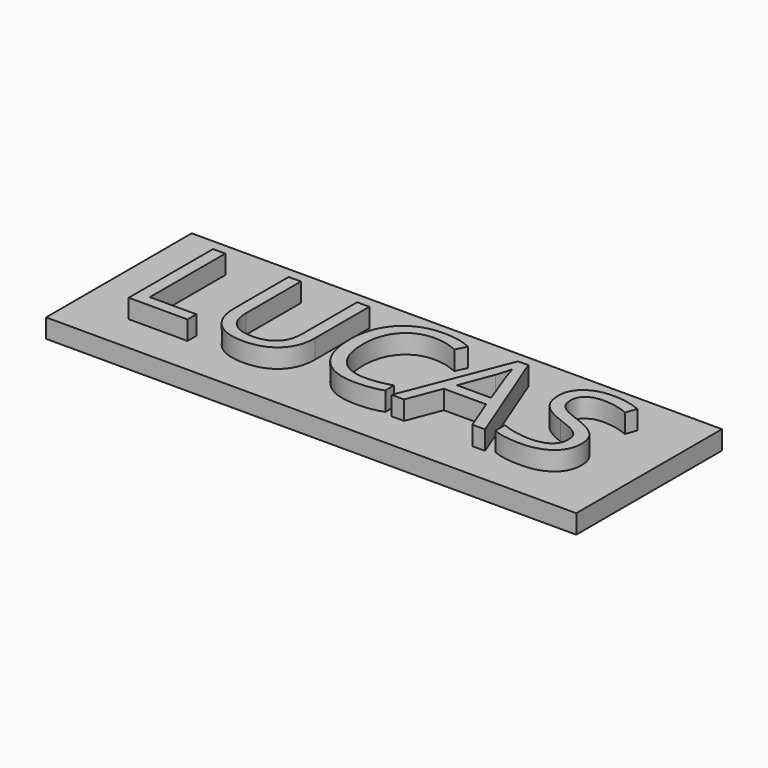
from build123d import *

# Parameters (mm, degrees)
F0_TEXT_SIZE = 24.7679024886
F1_DEPTH     = 6.35
F0_W         = 88.9
F0_H         = 30.5308
F2_DEPTH     = 3.175


# Not quite as in the source:
# - Text() gives the source's letters only with a copy of the font that has no kerning and outlines rounded to 1/6400 em; it was checked with that copy


with BuildPart() as f1:
    # F0 (on Top) → F1 (new body)
    with BuildSketch(Plane.XY):
        with Locations((0, -17.8328897918)):
            Text('LUCAS', F0_TEXT_SIZE, font='Open Sans', text_align=(TextAlign.LEFT, TextAlign.BOTTOM))
    extrude(amount=F1_DEPTH)


with BuildPart() as f2:
    # F0 (on Top) → F2 (new body)
    with BuildSketch(Plane.XY):
        with Locations((38.1, -8.9154)):
            Rectangle(F0_W, F0_H)
        Polygon((12.2872016252, -17.8328897918), (2.4303504317, -17.8328897918), (2.4303504317, -0.1509294058), (4.4853123413, -0.1509294058), (4.4853123413, -15.9714271204), (12.2872016252, -15.9714271204), align=None, mode=Mode.SUBTRACT)
        with BuildLine():
            Line((26.5829253428, -0.1509294058), (28.6378872524, -0.1509294058))
            Line((28.6378872524, -0.1509294058), (28.6378872524, -11.5906043677))
            add(Edge.make_bspline(
                [(28.6378872524, -11.5906043677), (28.6378872524, -14.616932453), (26.8112544439, -16.3468156425)],
                knots=[0, 0, 0, 1, 1, 1], degree=2))
            add(Edge.make_bspline(
                [(26.8112544439, -16.3468156425), (24.9846216353, -18.0766988319), (21.7918842052, -18.0766988319)],
                knots=[0, 0, 0, 1, 1, 1], degree=2))
            add(Edge.make_bspline(
                [(21.7918842052, -18.0766988319), (18.599146775, -18.0766988319), (16.8518486541, -16.3332706958)],
                knots=[0, 0, 0, 1, 1, 1], degree=2))
            add(Edge.make_bspline(
                [(16.8518486541, -16.3332706958), (15.1045505333, -14.5898425597), (15.1045505333, -11.5441645505)],
                knots=[0, 0, 0, 1, 1, 1], degree=2))
            Line((15.1045505333, -11.5441645505), (15.1045505333, -0.1509294058))
            Line((15.1045505333, -0.1509294058), (17.1633824276, -0.1509294058))
            Line((17.1633824276, -0.1509294058), (17.1633824276, -11.6873539868))
            add(Edge.make_bspline(
                [(17.1633824276, -11.6873539868), (17.1633824276, -13.9009852717), (18.3727526663, -15.0871356018)],
                knots=[0, 0, 0, 1, 1, 1], degree=2))
            add(Edge.make_bspline(
                [(18.3727526663, -15.0871356018), (19.582122905, -16.2732859319), (21.9273336719, -16.2732859319)],
                knots=[0, 0, 0, 1, 1, 1], degree=2))
            add(Edge.make_bspline(
                [(21.9273336719, -16.2732859319), (24.1641848654, -16.2732859319), (25.3735551041, -15.0813306247)],
                knots=[0, 0, 0, 1, 1, 1], degree=2))
            add(Edge.make_bspline(
                [(25.3735551041, -15.0813306247), (26.5829253428, -13.8893753174), (26.5829253428, -11.6641340782)],
                knots=[0, 0, 0, 1, 1, 1], degree=2))
            Line((26.5829253428, -11.6641340782), (26.5829253428, -0.1509294058))
        make_face(mode=Mode.SUBTRACT)
        with BuildLine():
            add(Edge.make_bspline(
                [(44.9034332148, -2.6780294566), (42.8949111224, -1.737623159), (40.88638903, -1.737623159)],
                knots=[0, 0, 0, 1, 1, 1], degree=2))
            add(Edge.make_bspline(
                [(40.88638903, -1.737623159), (37.9722905028, -1.737623159), (36.2849771458, -3.678420518)],
                knots=[0, 0, 0, 1, 1, 1], degree=2))
            add(Edge.make_bspline(
                [(36.2849771458, -3.678420518), (34.5976637887, -5.6192178771), (34.5976637887, -8.9938445912)],
                knots=[0, 0, 0, 1, 1, 1], degree=2))
            add(Edge.make_bspline(
                [(34.5976637887, -8.9938445912), (34.5976637887, -12.4613509396), (36.2249923819, -14.3557084815)],
                knots=[0, 0, 0, 1, 1, 1], degree=2))
            add(Edge.make_bspline(
                [(36.2249923819, -14.3557084815), (37.8523209751, -16.2500660234), (40.8631691214, -16.2500660234)],
                knots=[0, 0, 0, 1, 1, 1], degree=2))
            add(Edge.make_bspline(
                [(40.8631691214, -16.2500660234), (42.7130218385, -16.2500660234), (45.0853224987, -15.584428644)],
                knots=[0, 0, 0, 1, 1, 1], degree=2))
            Line((45.0853224987, -15.584428644), (45.0853224987, -17.3839715592))
            add(Edge.make_bspline(
                [(45.0853224987, -17.3839715592), (43.2470797359, -18.0766988319), (40.5497003555, -18.0766988319)],
                knots=[0, 0, 0, 1, 1, 1], degree=2))
            add(Edge.make_bspline(
                [(40.5497003555, -18.0766988319), (36.6448857288, -18.0766988319), (34.5221990858, -15.7043981717)],
                knots=[0, 0, 0, 1, 1, 1], degree=2))
            add(Edge.make_bspline(
                [(34.5221990858, -15.7043981717), (32.3995124429, -13.3320975114), (32.3995124429, -8.9667546978)],
                knots=[0, 0, 0, 1, 1, 1], degree=2))
            add(Edge.make_bspline(
                [(32.3995124429, -8.9667546978), (32.3995124429, -6.2345454545), (33.4211884205, -4.1795835449)],
                knots=[0, 0, 0, 1, 1, 1], degree=2))
            add(Edge.make_bspline(
                [(33.4211884205, -4.1795835449), (34.4428643982, -2.1246216353), (36.3720518029, -1.0120010157)],
                knots=[0, 0, 0, 1, 1, 1], degree=2))
            add(Edge.make_bspline(
                [(36.3720518029, -1.0120010157), (38.3012392077, 0.1006196039), (40.9134789233, 0.1006196039)],
                knots=[0, 0, 0, 1, 1, 1], degree=2))
            add(Edge.make_bspline(
                [(40.9134789233, 0.1006196039), (43.6921279837, 0.1006196039), (45.7741797867, -0.9133164043)],
                knots=[0, 0, 0, 1, 1, 1], degree=2))
            Line((45.7741797867, -0.9133164043), (44.9034332148, -2.6780294566))
        make_face(mode=Mode.SUBTRACT)
        Polygon((62.1867851701, -17.8328897918), (60.05829355, -17.8328897918), (57.8562722194, -12.2098019299), (50.7703301168, -12.2098019299), (48.5953986795, -17.8328897918), (46.5133468766, -17.8328897918), (53.5025393601, -0.0773996953), (55.2324225495, -0.0773996953), align=None, mode=Mode.SUBTRACT)
        with BuildLine():
            add(Edge.make_bspline(
                [(73.5490604368, -10.1780599289), (74.593956323, -11.3158354495), (74.593956323, -13.1269883189)],
                knots=[0, 0, 0, 1, 1, 1], degree=2))
            add(Edge.make_bspline(
                [(74.593956323, -13.1269883189), (74.593956323, -15.4605891315), (72.9008379888, -16.7686439817)],
                knots=[0, 0, 0, 1, 1, 1], degree=2))
            add(Edge.make_bspline(
                [(72.9008379888, -16.7686439817), (71.2077196546, -18.0766988319), (68.3052310818, -18.0766988319)],
                knots=[0, 0, 0, 1, 1, 1], degree=2))
            add(Edge.make_bspline(
                [(68.3052310818, -18.0766988319), (65.1628034535, -18.0766988319), (63.467750127, -17.2640020315)],
                knots=[0, 0, 0, 1, 1, 1], degree=2))
            Line((63.467750127, -17.2640020315), (63.467750127, -15.2825698324))
            add(Edge.make_bspline(
                [(63.467750127, -15.2825698324), (64.5590858304, -15.7392280345), (65.8400507872, -16.0062569832)],
                knots=[0, 0, 0, 1, 1, 1], degree=2))
            add(Edge.make_bspline(
                [(65.8400507872, -16.0062569832), (67.121015744, -16.2732859319), (68.3787607923, -16.2732859319)],
                knots=[0, 0, 0, 1, 1, 1], degree=2))
            add(Edge.make_bspline(
                [(68.3787607923, -16.2732859319), (70.4337227019, -16.2732859319), (71.4747486034, -15.493484002)],
                knots=[0, 0, 0, 1, 1, 1], degree=2))
            add(Edge.make_bspline(
                [(71.4747486034, -15.493484002), (72.5157745048, -14.7136820721), (72.5157745048, -13.3204875571)],
                knots=[0, 0, 0, 1, 1, 1], degree=2))
            add(Edge.make_bspline(
                [(72.5157745048, -13.3204875571), (72.5157745048, -12.4033011681), (72.1461909599, -11.8169984764)],
                knots=[0, 0, 0, 1, 1, 1], degree=2))
            add(Edge.make_bspline(
                [(72.1461909599, -11.8169984764), (71.7766074149, -11.2306957847), (70.9116658202, -10.7334027425)],
                knots=[0, 0, 0, 1, 1, 1], degree=2))
            add(Edge.make_bspline(
                [(70.9116658202, -10.7334027425), (70.0467242255, -10.2361097004), (68.2820111732, -9.6091721686)],
                knots=[0, 0, 0, 1, 1, 1], degree=2))
            add(Edge.make_bspline(
                [(68.2820111732, -9.6091721686), (65.8168308786, -8.7268156425), (64.7583900457, -7.5174454038)],
                knots=[0, 0, 0, 1, 1, 1], degree=2))
            add(Edge.make_bspline(
                [(64.7583900457, -7.5174454038), (63.6999492128, -6.3080751651), (63.6999492128, -4.3614728288)],
                knots=[0, 0, 0, 1, 1, 1], degree=2))
            add(Edge.make_bspline(
                [(63.6999492128, -4.3614728288), (63.6999492128, -2.3181208735), (65.2343981717, -1.1087506348)],
                knots=[0, 0, 0, 1, 1, 1], degree=2))
            add(Edge.make_bspline(
                [(65.2343981717, -1.1087506348), (66.7688471305, 0.1006196039), (69.2998171661, 0.1006196039)],
                knots=[0, 0, 0, 1, 1, 1], degree=2))
            add(Edge.make_bspline(
                [(69.2998171661, 0.1006196039), (71.9352767902, 0.1006196039), (74.1489080752, -0.8668765871)],
                knots=[0, 0, 0, 1, 1, 1], degree=2))
            Line((74.1489080752, -0.8668765871), (73.5064906044, -2.654809548))
            add(Edge.make_bspline(
                [(73.5064906044, -2.654809548), (71.316079228, -1.737623159), (69.2495073641, -1.737623159)],
                knots=[0, 0, 0, 1, 1, 1], degree=2))
            add(Edge.make_bspline(
                [(69.2495073641, -1.737623159), (67.6163737938, -1.737623159), (66.6972524124, -2.4380904012)],
                knots=[0, 0, 0, 1, 1, 1], degree=2))
            add(Edge.make_bspline(
                [(66.6972524124, -2.4380904012), (65.778131031, -3.1385576435), (65.778131031, -4.3846927374)],
                knots=[0, 0, 0, 1, 1, 1], degree=2))
            add(Edge.make_bspline(
                [(65.778131031, -4.3846927374), (65.778131031, -5.3018791265), (66.1167546978, -5.8901168106)],
                knots=[0, 0, 0, 1, 1, 1], degree=2))
            add(Edge.make_bspline(
                [(66.1167546978, -5.8901168106), (66.4553783647, -6.4783544947), (67.2603351955, -6.9679075673)],
                knots=[0, 0, 0, 1, 1, 1], degree=2))
            add(Edge.make_bspline(
                [(67.2603351955, -6.9679075673), (68.0652920264, -7.4574606399), (69.7216455053, -8.0495683088)],
                knots=[0, 0, 0, 1, 1, 1], degree=2))
            add(Edge.make_bspline(
                [(69.7216455053, -8.0495683088), (72.5041645505, -9.0402844083), (73.5490604368, -10.1780599289)],
                knots=[0, 0, 0, 1, 1, 1], degree=2))
        make_face(mode=Mode.SUBTRACT)
    extrude(amount=F2_DEPTH)


with BuildPart() as f2b:
    # F0 (on Top) → F2, piece 2 (new body)
    with BuildSketch(Plane.XY):
        with BuildLine():
            Line((51.4978872524, -10.3599492128), (57.2177247334, -10.3599492128))
            Line((57.2177247334, -10.3599492128), (55.158892839, -4.8800507872))
            add(Edge.make_bspline(
                [(55.158892839, -4.8800507872), (54.7602844083, -3.8390248857), (54.3384560691, -2.3297308278)],
                knots=[0, 0, 0, 1, 1, 1], degree=2))
            add(Edge.make_bspline(
                [(54.3384560691, -2.3297308278), (54.0714271204, -3.490726257), (53.5760690706, -4.8800507872)],
                knots=[0, 0, 0, 1, 1, 1], degree=2))
            Line((53.5760690706, -4.8800507872), (51.4978872524, -10.3599492128))
        make_face()
    extrude(amount=F2_DEPTH)


solid = Compound([f1.part, f2.part, f2b.part])
